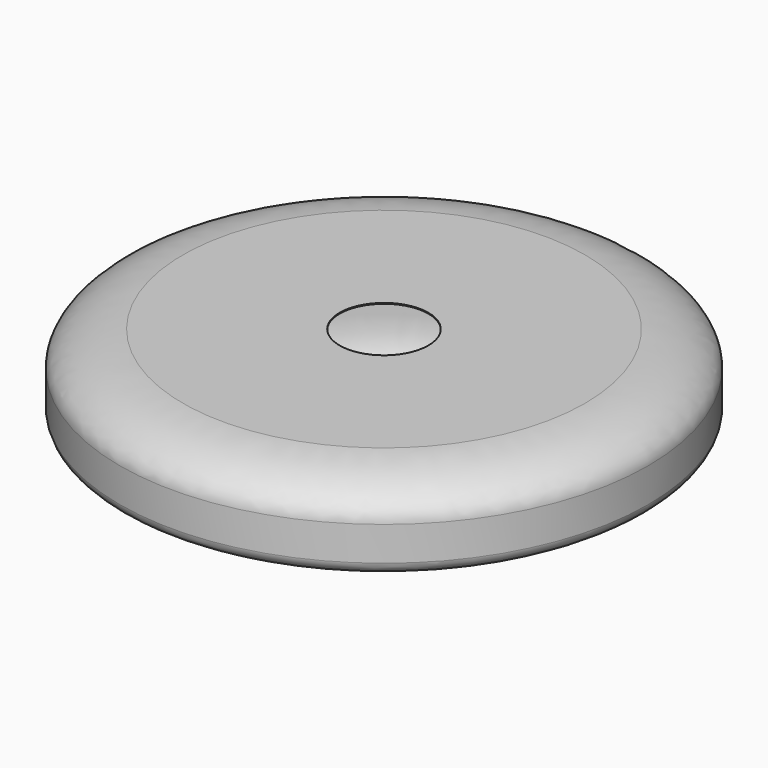
from build123d import *

# Parameters (mm, degrees)
F5_COPIES_COUNT = 50


# Not quite as in the source:
# - a pattern or mirror of a feature is missing from the dataset's text; its kind, count and spacing are read off the source's solid


with BuildPart() as f1:
    # F0 (on Front) → F1 (revolve)
    with BuildSketch(Plane.XZ):
        with BuildLine():
            add(Edge.make_bspline(
                [(148.6038176, 0.5235271343), (169.5855765746, 0), (195.9310880566, -10.7523894855), (195.9310880566, -25.4327541639)],
                knots=[0, 0, 0, 0, 53.9777645675, 53.9777645675, 53.9777645675, 53.9777645675], degree=3))
            Line((195.9310880566, -25.4327541639), (195.9310880566, -48.2927541639))
            add(Edge.make_bspline(
                [(195.9310880566, -48.2927541639), (195.8497955065, -56.6788213958), (168.7218850718, -72.0750381267), (82.5055381298, -42.6369075131), (43.2103020851, -133.3847761654), (31.75, -91.0328907508)],
                knots=[0, 0, 0, 0, 0.2377208586, 0.6722431183, 1, 1, 1, 1], degree=3))
            Line((31.75, -91.0328907508), (31.75, -91.6678907508))
            add(Edge.make_bspline(
                [(31.75, -91.6678907508), (42.5060250758, -134.880737854), (83.0978962555, -43.5490425098), (168.3266424363, -72.0878412276), (196.0189313024, -56.8945984297), (196.5660880566, -49.906556933)],
                knots=[0, 0, 0, 0, 0.3277269105, 0.7629447746, 1, 1, 1, 1], degree=3))
            Line((196.5660880566, -49.906556933), (196.5660880566, -24.506556933))
            add(Edge.make_bspline(
                [(196.5660880566, -24.506556933), (196.5660880566, -9.7524957803), (169.4746922507, 1.1585271343), (149.6336606, 1.1585271343)],
                knots=[0, 0, 0, 0, 53.4915814605, 53.4915814605, 53.4915814605, 53.4915814605], degree=3))
            Line((149.6336606, 1.1585271343), (33.02, 1.1585271343))
            Line((33.02, 1.1585271343), (33.02, 0.5235271343))
            Line((33.02, 0.5235271343), (148.6038176, 0.5235271343))
        make_face()
    revolve(axis=Axis((0, 0, -47.6807364329), (0, 0, -1)))

    # F4 (on face) → F5 (join, up to the next surface of F1)
    with BuildSketch(Plane(origin=(-127.5196369192, -127.5196369192, 0), x_dir=(0.7071067812, -0.7071067812, 0), z_dir=(-0.7071067812, -0.7071067812, 0))):
        with BuildLine():
            add(Edge.make_bspline(
                [(71.806074389, -39.4999235868), (71.5646540911, -47.6975520405), (72.5949747162, -51.4410332824), (63.4895045581, -55.3561263385), (52.8522965393, -57.3901794851)],
                knots=[0, 0, 0, 0, 0.4401357027, 1, 1, 1, 1], degree=3))
            Line((71.806074389, -39.4999235868), (71.1371566841, -39.4999235868))
            ThreePointArc((71.1371566841, -39.4999235868), (67.4416529048, -41.0942885203), (66.0658269354, -44.8765960998))
            add(Edge.make_bspline(
                [(66.0658269354, -44.8765960998), (66.171727548, -46.6868646744), (66.7689525826, -51.3972943975), (60.8864146443, -51.2559585148), (57.3228179978, -51.6866156404)],
                knots=[0.2470779886, 0.2470779886, 0.2470779886, 0.2470779886, 0.46732984, 0.8354827954, 0.8354827954, 0.8354827954, 0.8354827954], degree=3))
            ThreePointArc((57.3228179978, -51.6866156404), (54.130813211, -53.3601851267), (52.8522965393, -56.7299216897))
            Line((52.8522965393, -56.7299216897), (52.8522965393, -57.3901794851))
        make_face()
    f5 = extrude(until=Until.NEXT)

    # F5_copies: F5 ×50 about axis
    f5_copies_axis = Axis((0, 0, 0), (0, 0, 1))
    for i in range(1, F5_COPIES_COUNT):
        add(f5.rotate(f5_copies_axis, i * 360 / F5_COPIES_COUNT))


solid = f1.part
